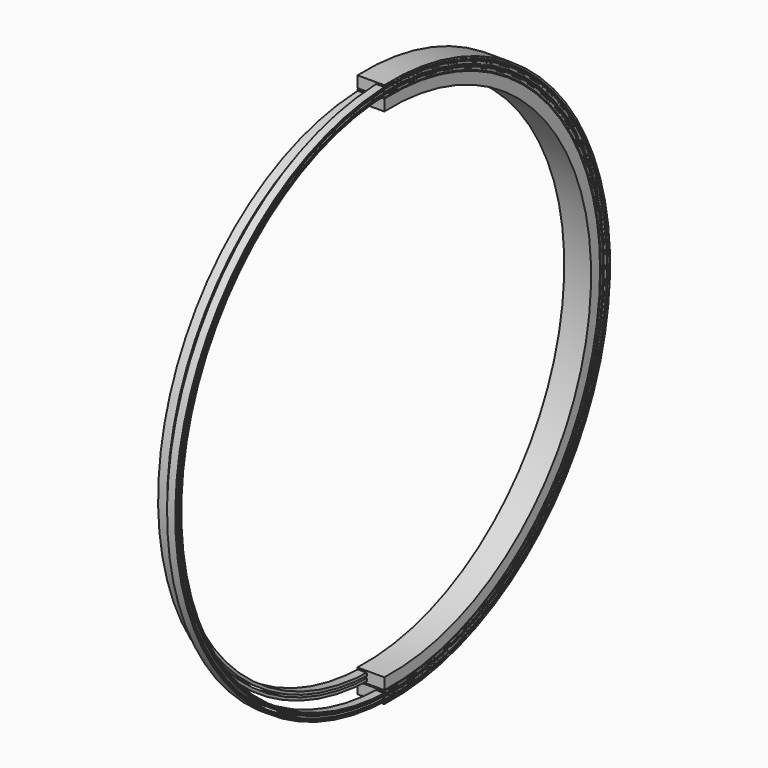
from build123d import *

# Parameters (mm, degrees)
F5_W      = 591.8968357146
F5_H      = 1187.1953699738
F6_DEPTH  = 127
F9_W      = 733.9637354016
F9_H      = 1242.4891926348
F10_DEPTH = 76.2


with BuildPart() as f3:
    # F0 (on Front) → F3 (revolve)
    with BuildSketch(Plane.XZ):
        Polygon((38.1000004709, 26.8875419878), (-20.9550000727, 26.8875419878), (-20.9550000727, 23.0716671795), (0, 23.0716671795), (0, 16.0866659135), (-20.7433328032, 16.0866659135), (-20.7433328032, 12.4883335084), (0, 12.4883335084), (0, 5.7150004432), (-20.5316673964, 5.7150004432), (-20.5316673964, 2.1166666411), (38.1000004709, 2.1166666411), align=None)
    revolve(axis=Axis((60.2579116821, 0, 575.2654075623), (1, 0, 0)))

    # F5 (on Right) → F6 (cut, symmetric)
    with BuildSketch(Plane.YZ):
        with Locations((-316.3586538285, 570.1241148636)):
            Rectangle(F5_W, F5_H)
    extrude(amount=F6_DEPTH, both=True, mode=Mode.SUBTRACT)


with BuildPart() as f4:
    # F2 (on Front) → F4 (revolve)
    with BuildSketch(Plane.XZ):
        Polygon((-0.6466466002, 22.5789006799), (-20.6548310816, 22.5789006799), (-20.6548310816, 20.1677661389), (-2.7616769075, 20.1677661389), (-2.7616769075, 18.6449438334), (-20.6548310816, 18.6449438334), (-20.6548310816, 16.6145153344), (-0.6466466002, 16.6145153344), align=None)
    revolve(axis=Axis((60.2579116821, 0, 575.2654075623), (1, 0, 0)))


with BuildPart() as f4b:
    # F2 (on Front) → F4, piece 2 (revolve)
    with BuildSketch(Plane.XZ):
        Polygon((-0.6466466002, 12.0339053683), (-20.6548310816, 12.0339053683), (-20.6548310816, 9.6227708273), (-2.7616769075, 9.6227708273), (-2.7616769075, 8.0999485217), (-20.6548310816, 8.0999485217), (-20.6548310816, 6.0695200227), (-0.6466466002, 6.0695200227), align=None)
    revolve(axis=Axis((60.2579116821, 0, 575.2654075623), (1, 0, 0)))


with BuildPart() as f8:
    # F7 (on Front) → F8 (revolve)
    with BuildSketch(Plane.XZ):
        Polygon((38.3181218058, 0.132874471), (-20.2347189479, 0.132874471), (-20.2347189479, -24.6380008757), (38.6671647429, -24.6380008757), (38.6671647429, -21.0396670736), (19.6266453713, -21.0396670736), (19.6266453713, -14.2663340084), (38.2877346128, -14.2663340084), (38.2877346128, -10.6680016033), (19.4588676095, -10.6680016033), (19.4588676095, -3.6830003373), (38.3181218058, -3.6830003373), align=None)
    revolve(axis=Axis((60.2579116821, 0, 575.2654075623), (1, 0, 0)))

    # F9 (on Right) → F10 (cut, symmetric)
    with BuildSketch(Plane.YZ):
        with Locations((-388.1385289133, 595.0256120414)):
            Rectangle(F9_W, F9_H)
    extrude(amount=F10_DEPTH, both=True, mode=Mode.SUBTRACT)


with BuildPart() as f12:
    # F11 (on Front) → F12 (revolve)
    with BuildSketch(Plane.XZ):
        Polygon((38.3636948536, -3.8806593511), (20.1826238772, -3.8806593511), (20.1826238772, -9.8450446967), (38.3437645651, -9.8450446967), (38.3437645651, -7.8146161977), (23.0500668986, -7.8146161977), (23.0500668986, -6.2917938922), (38.3636948536, -6.2917938922), align=None)
    revolve(axis=Axis((60.2579116821, 0, 575.2654075623), (1, 0, 0)))


with BuildPart() as f12b:
    # F11 (on Front) → F12, piece 2 (revolve)
    with BuildSketch(Plane.XZ):
        Polygon((38.3437645651, -14.4256546628), (20.1826238772, -14.4256546628), (20.1826238772, -20.3900400084), (38.3636948536, -20.3900400084), (38.3636948536, -18.3596115094), (23.0500687612, -18.3596115094), (23.0500687612, -16.8367892038), (38.3437645651, -16.8367892038), align=None)
    revolve(axis=Axis((60.2579116821, 0, 575.2654075623), (1, 0, 0)))


solid = Compound([f3.part, f4.part, f4b.part, f8.part, f12.part, f12b.part])
